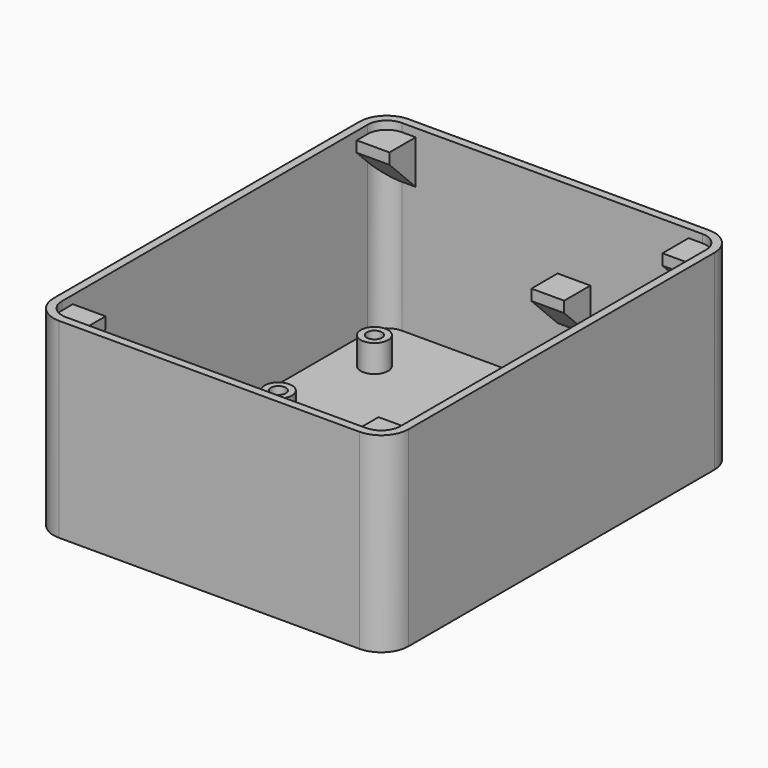
from build123d import *

# Parameters (mm, degrees)
F0_W      = 65
F0_H      = 80
F1_DEPTH  = 35
F2_R      = 5
F3_T      = -1.5
F6_DEPTH  = 8
F7_R      = 2.5
F7_R_2    = 1.375
F9_DEPTH  = 5
F10_W     = 6
F10_H     = 7.5
F11_DEPTH = 8
F12_SIZE  = 5.99999


# Not quite as in the source:
# - a fillet or chamfer is up to 0.001 mm smaller than in the source, because OpenCascade refuses the exact size


with BuildPart() as f1:
    # F0 (on Top) → F1 (new body)
    with BuildSketch(Plane.XY):
        with Locations((1.2058935761, -13.8313528726)):
            Rectangle(F0_W, F0_H)
    extrude(amount=F1_DEPTH)

    # F2
    f2_edges = [f1.edges().sort_by_distance(p)[0] for p in [
        (-31.294106, -53.831353, 17.5),
        (-31.294106, 26.168647, 17.5),
        (33.705894, -53.831353, 17.5),
        (33.705894, 26.168647, 17.5),
    ]]
    fillet(f2_edges, radius=F2_R)

    # F3
    f3_openings = [f1.faces().sort_by_distance(p)[0] for p in [
        (1.205894, -13.831353, 35),
    ]]
    offset(amount=F3_T, openings=f3_openings)

    # F5 (on offset) → F6 (join)
    with BuildSketch(Plane.XY.offset(33.5)):
        with BuildLine():
            Line((-29.7941064239, 18.6686471274), (-23.7941064239, 18.6686471274))
            Line((-23.7941064239, 18.6686471274), (-23.7941064239, 24.6686471274))
            Line((-23.7941064239, 24.6686471274), (-26.2941064239, 24.6686471274))
            ThreePointArc((-26.2941064239, 24.6686471274), (-28.768980158, 23.6435208615), (-29.7941064239, 21.1686471274))
            Line((-29.7941064239, 21.1686471274), (-29.7941064239, 18.6686471274))
        make_face()
        with BuildLine():
            Line((28.7058935761, 24.6686471274), (26.2058935761, 24.6686471274))
            Line((26.2058935761, 24.6686471274), (26.2058935761, 18.6686471274))
            Line((26.2058935761, 18.6686471274), (32.2058935761, 18.6686471274))
            Line((32.2058935761, 18.6686471274), (32.2058935761, 21.1686471274))
            ThreePointArc((32.2058935761, 21.1686471274), (31.1807673103, 23.6435208615), (28.7058935761, 24.6686471274))
        make_face()
        with BuildLine():
            Line((26.2058935761, -46.3313528726), (26.2058935761, -52.3313528726))
            Line((26.2058935761, -52.3313528726), (28.7058935761, -52.3313528726))
            ThreePointArc((28.7058935761, -52.3313528726), (31.1807673103, -51.3062266068), (32.2058935761, -48.8313528726))
            Line((32.2058935761, -48.8313528726), (32.2058935761, -46.3313528726))
            Line((32.2058935761, -46.3313528726), (26.2058935761, -46.3313528726))
        make_face()
        with BuildLine():
            Line((-23.7941064239, -46.3313528726), (-29.7941064239, -46.3313528726))
            Line((-29.7941064239, -46.3313528726), (-29.7941064239, -48.8313528726))
            ThreePointArc((-29.7941064239, -48.8313528726), (-28.768980158, -51.3062266068), (-26.2941064239, -52.3313528726))
            Line((-26.2941064239, -52.3313528726), (-23.7941064239, -52.3313528726))
            Line((-23.7941064239, -52.3313528726), (-23.7941064239, -46.3313528726))
        make_face()
    extrude(amount=-F6_DEPTH)

    # F7 (on face) → F9 (join)
    with BuildSketch(Plane.XY.offset(1.5)):
        with Locations((-22.5441064239, 13.6686471274)):
            Circle(F7_R)
        with Locations((-22.5441064239, 13.6686471274)):
            Circle(F7_R_2, mode=Mode.SUBTRACT)
        with Locations((-22.5441064239, -8.3313528726)):
            Circle(F7_R)
        with Locations((-22.5441064239, -8.3313528726)):
            Circle(F7_R_2, mode=Mode.SUBTRACT)
        with Locations((24.9558935761, 13.6686471274)):
            Circle(F7_R)
        with Locations((24.9558935761, 13.6686471274)):
            Circle(F7_R_2, mode=Mode.SUBTRACT)
        with Locations((24.9558935761, -8.3313528726)):
            Circle(F7_R)
        with Locations((24.9558935761, -8.3313528726)):
            Circle(F7_R_2, mode=Mode.SUBTRACT)
        with BuildLine():
            Line((17.2198255986, -40.3313528726), (21.6919615536, -40.3313528726))
            ThreePointArc((21.6919615536, -40.3313528726), (22.258410653, -39.4018191419), (22.4558935761, -38.3313528726))
            ThreePointArc((22.4558935761, -38.3313528726), (18.3854273068, -35.5288357957), (17.2198255986, -40.3313528726))
        make_face()
        with BuildLine():
            ThreePointArc((-14.0441064239, -38.3313528726), (-18.1145726932, -35.5288357957), (-19.2801744014, -40.3313528726))
            Line((-19.2801744014, -40.3313528726), (-14.8080384464, -40.3313528726))
            ThreePointArc((-14.8080384464, -40.3313528726), (-14.241589347, -39.4018191419), (-14.0441064239, -38.3313528726))
        make_face()
    extrude(amount=F9_DEPTH)

    # F10 (on offset) → F11 (join)
    with BuildSketch(Plane.XY.offset(20)):
        with Locations((5.2058935761, 22.4186471274)):
            Rectangle(F10_W, F10_H)
        with BuildLine():
            Line((26.2058935761, 18.6686471274), (32.2058935761, 18.6686471274))
            Line((32.2058935761, 18.6686471274), (32.2058935761, 21.1686471274))
            ThreePointArc((32.2058935761, 21.1686471274), (31.1807673103, 23.6435208615), (28.7058935761, 24.6686471274))
            Line((28.7058935761, 24.6686471274), (26.2058935761, 24.6686471274))
            Line((26.2058935761, 24.6686471274), (26.2058935761, 18.6686471274))
        make_face()
        with BuildLine():
            Line((32.2058935761, -46.3313528726), (26.2058935761, -46.3313528726))
            Line((26.2058935761, -46.3313528726), (26.2058935761, -52.3313528726))
            Line((26.2058935761, -52.3313528726), (28.7058935761, -52.3313528726))
            ThreePointArc((28.7058935761, -52.3313528726), (31.1807673103, -51.3062266068), (32.2058935761, -48.8313528726))
            Line((32.2058935761, -48.8313528726), (32.2058935761, -46.3313528726))
        make_face()
        with Locations((5.2058935761, -50.0813528726)):
            Rectangle(F10_W, F10_H)
    extrude(amount=-F11_DEPTH)

    # F12 (size 6 in the source; OpenCascade refuses exactly that, so slightly less here)
    f12_edges = [f1.edges().sort_by_distance(p)[0] for p in [
        (29.205894, -46.331353, 25.5),
        (29.205894, -46.331353, 12),
        (5.205894, -46.331353, 12),
        (29.205894, 18.668647, 12),
        (29.205894, 18.668647, 25.5),
        (5.205894, 18.668647, 12),
        (-26.794106, 18.668647, 25.5),
        (-26.794106, -46.331353, 25.5),
    ]]
    chamfer(f12_edges, length=F12_SIZE)


solid = f1.part
